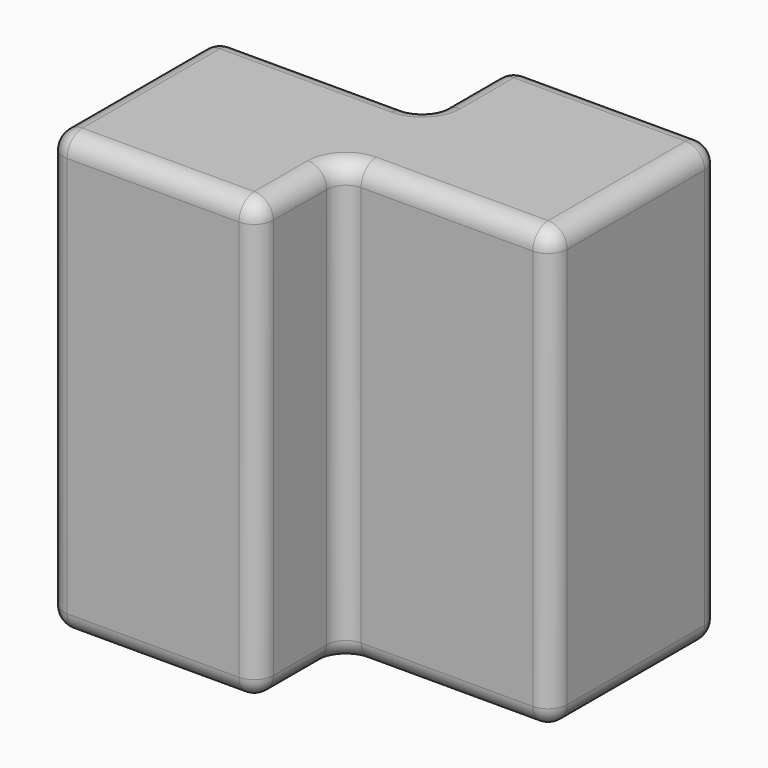
from build123d import *

# Parameters (mm, degrees)
F1_DEPTH = 146.05
F2_R     = 6.35


with BuildPart() as f1:
    # F0 (on Top) → F1 (new body)
    with BuildSketch(Plane.XY):
        Polygon((0, -52.3875), (0, -17.4625), (69.85, -17.4625), (69.85, 52.3875), (0, 52.3875), (0, 17.4625), (-69.85, 17.4625), (-69.85, -52.3875), align=None)
    extrude(amount=F1_DEPTH)

    # F2
    f2_edges = [f1.edges().sort_by_distance(p)[0] for p in [
        (-34.925, -52.3875, 146.05),
        (0, -34.925, 146.05),
        (34.925, -17.4625, 146.05),
        (69.85, 17.4625, 146.05),
        (34.925, 52.3875, 146.05),
        (0, 34.925, 146.05),
        (-34.925, 17.4625, 146.05),
        (-69.85, -17.4625, 146.05),
        (-69.85, -52.3875, 73.025),
        (0, -52.3875, 73.025),
        (-34.925, -52.3875, 0),
        (0, -17.4625, 73.025),
        (69.85, -17.4625, 73.025),
        (34.925, -17.4625, 0),
        (69.85, 52.3875, 73.025),
        (69.85, 17.4625, 0),
        (0, 52.3875, 73.025),
        (34.925, 52.3875, 0),
        (0, 17.4625, 73.025),
        (0, 34.925, 0),
        (-69.85, 17.4625, 73.025),
        (-34.925, 17.4625, 0),
        (-69.85, -17.4625, 0),
        (0, -34.925, 0),
    ]]
    fillet(f2_edges, radius=F2_R)


solid = f1.part
